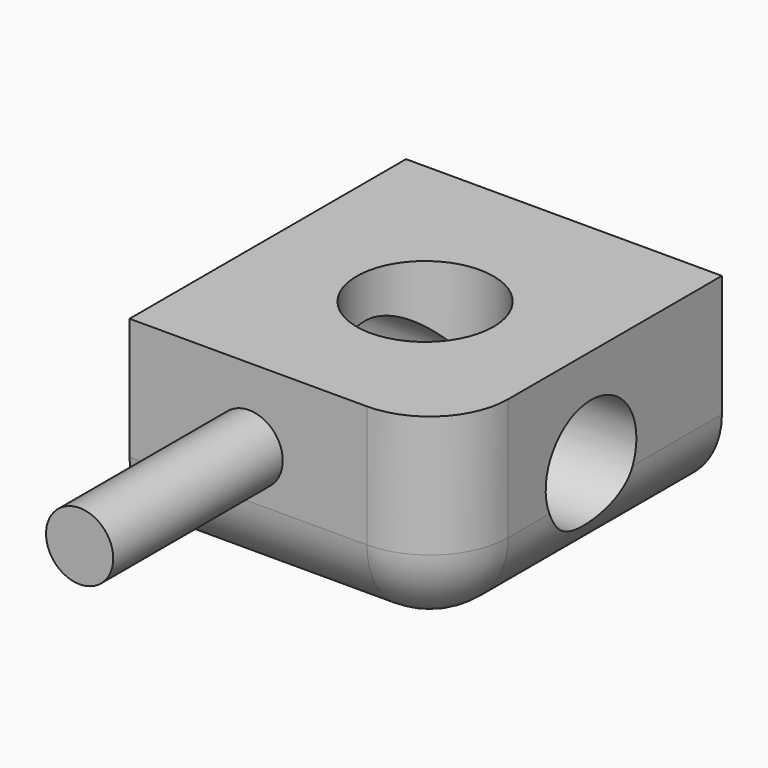
from build123d import *

# Parameters (mm, degrees)
F0_W         = 102.258592844
F0_H         = 64.8588836193
F1_DEPTH     = 111.87066
F2_R         = 22.1566524367
F3_DEPTH     = 123.47648
F4_R         = 18.3530030386
F5_DEPTH     = 205.67378
F6_T1_DEPTH  = 140.358592844
F6_T3_DEPTH  = 102.9588836193
F6_T5_DEPTH  = 149.97066
F6_S9_W      = 25.4
F6_S9_H      = 25.4
F6_T10_DEPTH = 25.4
F7_R         = 10.8823528673
F8_DEPTH     = 68.58648


# Not quite as in the source:
# - a fillet or chamfer that OpenCascade refuses, or shapes differently, is made with other operations: its cross-section is extruded or revolved along the edge and cut away or added


with BuildPart() as f1:
    # F0 (on Front) → F1 (new body)
    with BuildSketch(Plane.XZ):
        with Locations((51.129296422, 32.4294418097)):
            Rectangle(F0_W, F0_H)
    extrude(amount=F1_DEPTH)

    # F2 (on face) → F3 (cut)
    with BuildSketch(Plane.XY.offset(64.8588836193)):
        with Locations((52.4399839342, -57.8363165259)):
            Circle(F2_R)
    extrude(amount=-F3_DEPTH, mode=Mode.SUBTRACT)

    # F4 (on face) → F5 (cut)
    with BuildSketch(Plane.YZ.offset(102.258592844)):
        with Locations((-52.9614761472, 32.6913073659)):
            Circle(F4_R)
    extrude(amount=-F5_DEPTH, mode=Mode.SUBTRACT)

    # F6: fillet of radius 25.4 on 3 edges, made by hand

    # F6_s2 → F6_t1 (cut)
    with BuildSketch(Plane.YZ.offset(-63.5)):
        with BuildLine():
            ThreePointArc((-111.87066, 25.4), (-104.4311722421, 7.4394877579), (-86.47066, 0))
            Line((-86.47066, 0), (-111.87066, 0))
            Line((-111.87066, 0), (-111.87066, 25.4))
        make_face()
    extrude(amount=F6_T1_DEPTH, mode=Mode.SUBTRACT)

    # F6_s4 → F6_t3 (cut)
    with BuildSketch(Plane.XY.offset(25.4)):
        with BuildLine():
            ThreePointArc((76.858592844, -111.87066), (94.8191050861, -104.4311722421), (102.258592844, -86.47066))
            Line((102.258592844, -86.47066), (102.258592844, -111.87066))
            Line((102.258592844, -111.87066), (76.858592844, -111.87066))
        make_face()
    extrude(amount=F6_T3_DEPTH, mode=Mode.SUBTRACT)

    # F6_s6 → F6_t5 (cut)
    with BuildSketch(Plane.XZ.offset(-63.5)):
        with BuildLine():
            ThreePointArc((76.858592844, 0), (94.8191050861, 7.4394877579), (102.258592844, 25.4))
            Line((102.258592844, 25.4), (102.258592844, 0))
            Line((102.258592844, 0), (76.858592844, 0))
        make_face()
    extrude(amount=F6_T5_DEPTH, mode=Mode.SUBTRACT)


with BuildPart() as f6_tool8:
    # F6_s9 → F6_t10 (new body)
    with BuildSketch(Plane.XZ.offset(86.47066)):
        with Locations((89.558592844, 12.7)):
            Rectangle(F6_S9_W, F6_S9_H)
    extrude(amount=F6_T10_DEPTH)

    # F6_s11 → F6_t12 (revolve, cut)
    with BuildSketch(Plane(origin=(76.858592844, -86.47066, 25.4), x_dir=(-0.7071067812, 0, 0.7071067812), z_dir=(0.7071067812, 0, 0.7071067812))):
        with BuildLine():
            ThreePointArc((0, -25.4), (25.4, 0), (0, 25.4))
            Line((0, 25.4), (0, -25.4))
        make_face()
    revolve(axis=Axis((76.858592844, -86.47066, 25.4), (0, -1, 0)), mode=Mode.SUBTRACT)


with BuildPart() as f1_1:
    add(f1.part)

    # F6_t7: cut F6_tool8
    add(f6_tool8.part, mode=Mode.SUBTRACT)

    # F7 (on face) → F8 (join)
    with BuildSketch(Plane.XZ.offset(111.87066)):
        with Locations((38.7039594352, 40.518656373)):
            Circle(F7_R)
    extrude(amount=F8_DEPTH)


solid = f1_1.part
